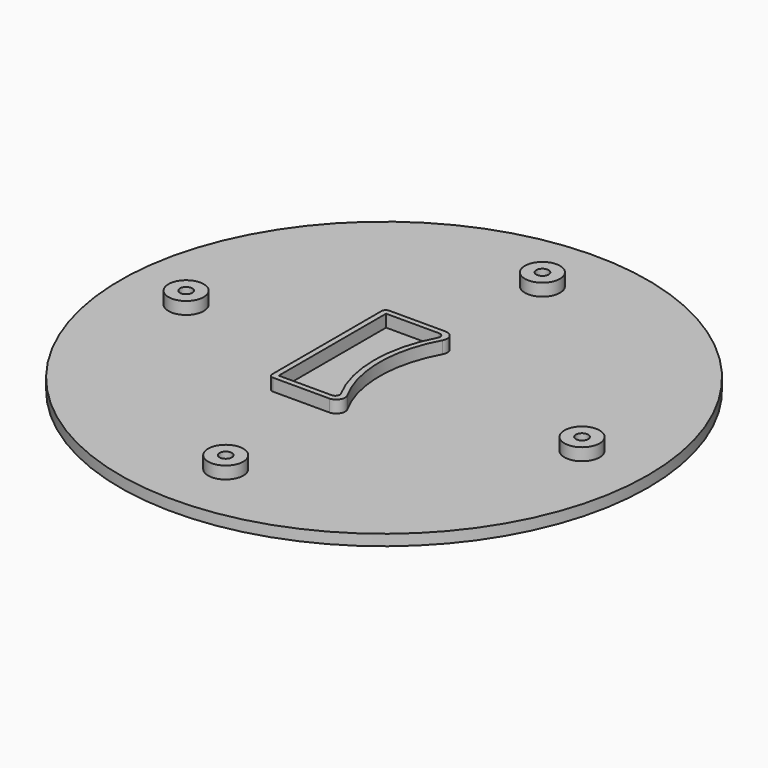
from build123d import *

# Parameters (mm, degrees)
F0_R     = 60
F1_DEPTH = 2.5
F2_R     = 1.4
F3_DEPTH = 12.5
F2_R_2   = 4
F4_DEPTH = 5.3
F6_DEPTH = 2.8
F7_R     = 2
F8_R     = 1


with BuildPart() as f1:
    # F0 (on Top) → F1 (new body)
    with BuildSketch(Plane.XY):
        Circle(F0_R)
    extrude(amount=F1_DEPTH)

    # F2 (on face) → F3 (cut, symmetric)
    with BuildSketch(Plane(origin=(0, 0, 0), x_dir=(1, 0, 0), z_dir=(0, 0, -1))):
        with Locations((0, -45)):
            Circle(F2_R)
        with Locations((-45, 0)):
            Circle(F2_R)
        with Locations((0, 45)):
            Circle(F2_R)
        with Locations((45, 0)):
            Circle(F2_R)
    extrude(amount=F3_DEPTH, both=True, mode=Mode.SUBTRACT)

    # F2 (on face) → F4 (join)
    with BuildSketch(Plane(origin=(0, 0, 0), x_dir=(1, 0, 0), z_dir=(0, 0, -1))):
        with Locations((-45, 0)):
            Circle(F2_R_2)
        with Locations((-45, 0)):
            Circle(F2_R, mode=Mode.SUBTRACT)
        with Locations((0, -45)):
            Circle(F2_R_2)
        with Locations((0, -45)):
            Circle(F2_R, mode=Mode.SUBTRACT)
        with Locations((45, 0)):
            Circle(F2_R_2)
        with Locations((45, 0)):
            Circle(F2_R, mode=Mode.SUBTRACT)
        with Locations((0, 45)):
            Circle(F2_R_2)
        with Locations((0, 45)):
            Circle(F2_R, mode=Mode.SUBTRACT)
    extrude(amount=-F4_DEPTH)

    # F5 (on face) → F6 (join)
    with BuildSketch(Plane.XY.offset(2.5)):
        with BuildLine():
            ThreePointArc((2.0400320513, 15.25), (2.4361318862, 15.8801411608), (2.8481367178, 16.5))
            Line((2.8481367178, 16.5), (-13, 16.5))
            Line((-13, 16.5), (-13, -16.5))
            Line((-13, -16.5), (2.8481367178, -16.5))
            ThreePointArc((2.8481367178, -16.5), (2.4361318862, -15.8801411608), (2.0400320513, -15.25))
            Line((2.0400320513, -15.25), (-11.75, -15.25))
            Line((-11.75, -15.25), (-11.75, 15.25))
            Line((-11.75, 15.25), (2.0400320513, 15.25))
        make_face()
        with BuildLine():
            ThreePointArc((3.5172935972, 15.25), (3.939229747, 15.8808335844), (4.3781079483, 16.5))
            Line((4.3781079483, 16.5), (2.8481367178, 16.5))
            ThreePointArc((2.8481367178, 16.5), (2.4361318862, 15.8801411608), (2.0400320513, 15.25))
            Line((2.0400320513, 15.25), (3.5172935972, 15.25))
        make_face()
        with BuildLine():
            Line((2.8481367178, -16.5), (4.3781079483, -16.5))
            ThreePointArc((4.3781079483, -16.5), (3.939229747, -15.8808335844), (3.5172935972, -15.25))
            Line((3.5172935972, -15.25), (2.0400320513, -15.25))
            ThreePointArc((2.0400320513, -15.25), (2.4361318862, -15.8801411608), (2.8481367178, -16.5))
        make_face()
        with BuildLine():
            ThreePointArc((3.5172935972, -15.25), (-1, 0), (3.5172935972, 15.25))
            Line((3.5172935972, 15.25), (2.0400320513, 15.25))
            ThreePointArc((2.0400320513, 15.25), (-2.25, 0), (2.0400320513, -15.25))
            Line((2.0400320513, -15.25), (3.5172935972, -15.25))
        make_face()
    extrude(amount=F6_DEPTH)

    # F7
    f7_edges = [f1.edges().sort_by_distance(p)[0] for p in [
        (4.378108, 16.5, 3.9),
        (4.378108, -16.5, 3.9),
    ]]
    fillet(f7_edges, radius=F7_R)

    # F8
    f8_edges = [f1.edges().sort_by_distance(p)[0] for p in [
        (2.040032, -15.25, 3.9),
        (2.040032, 15.25, 3.9),
        (-13, -16.5, 3.9),
        (-13, 16.5, 3.9),
    ]]
    fillet(f8_edges, radius=F8_R)


solid = f1.part
